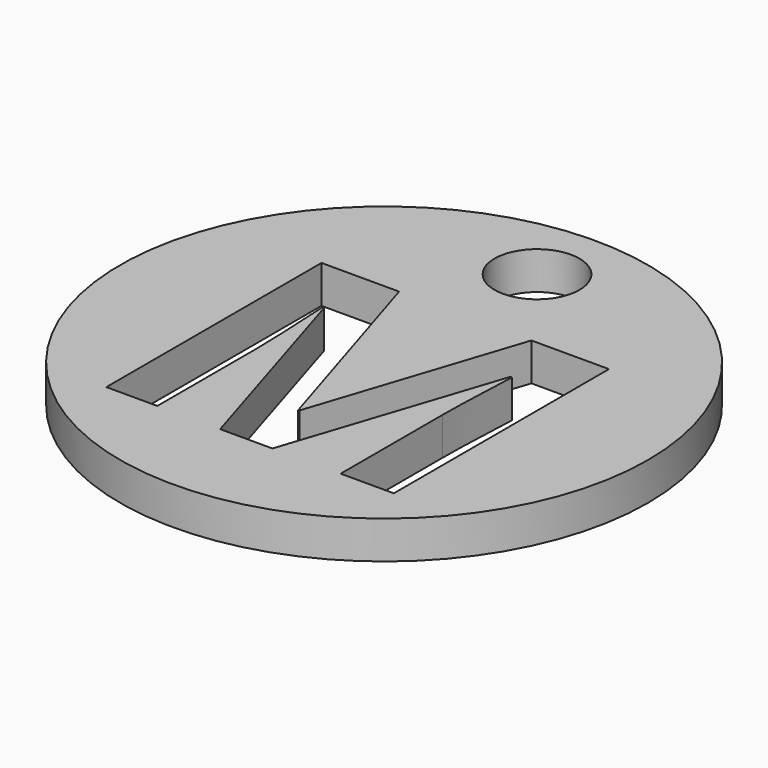
from build123d import *

# Parameters (mm, degrees)
F0_R         = 41.9250716585
F1_DEPTH     = 6
F2_R         = 6.7436301965
F3_DEPTH     = 71.2
F4_TEXT_SIZE = 59.8392992591
F5_DEPTH     = 14.3


# Not quite as in the source:
# - Text() gives the source's letters only with a copy of the font that has no kerning and outlines rounded to 1/6400 em; it was checked with that copy


with BuildPart() as f1:
    # F0 (on Top) → F1 (new body)
    with BuildSketch(Plane.XY):
        Circle(F0_R)
    extrude(amount=F1_DEPTH)

    # F2 (on Top) → F3 (cut)
    with BuildSketch(Plane.XY):
        with Locations((0, 30.3626079112)):
            Circle(F2_R)
    extrude(amount=F3_DEPTH, mode=Mode.SUBTRACT)

    # F4 (on Top) → F5 (cut)
    with BuildSketch(Plane.XY):
        with Locations((-28.1516183168, -26.680178009)):
            Text('M', F4_TEXT_SIZE, font='Open Sans', font_style=FontStyle.BOLD, text_align=(TextAlign.LEFT, TextAlign.BOTTOM))
    extrude(amount=F5_DEPTH, mode=Mode.SUBTRACT)


solid = f1.part
